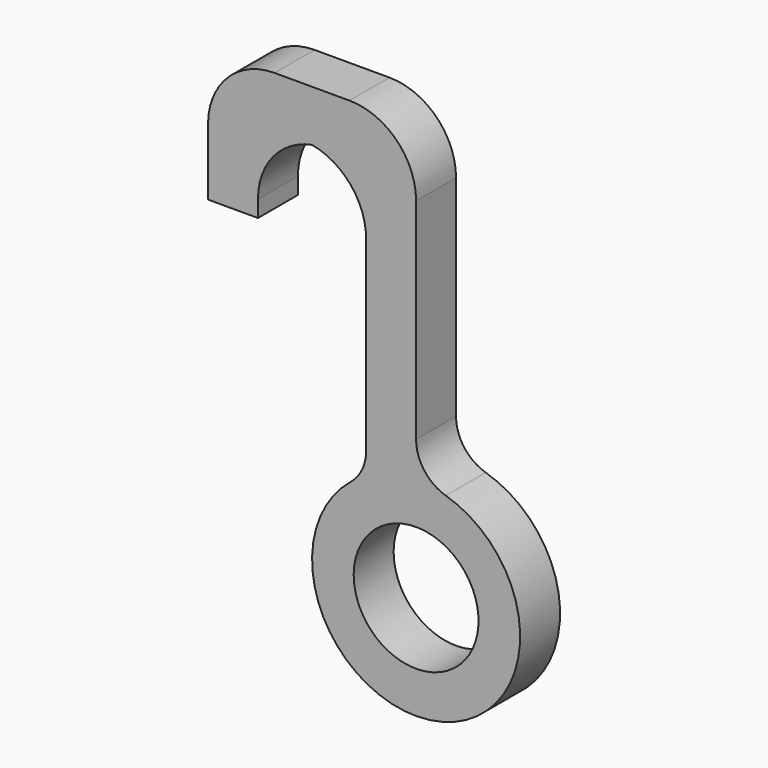
from build123d import *

# Parameters (mm, degrees)
F1_DEPTH    = 6
F2_R        = 12.5
F3_DEPTH    = 6
F5_D        = 15
F6_T1_DEPTH = 6
F6_T3_DEPTH = 46
F7_R        = 5


# Not quite as in the source:
# - a fillet or chamfer that OpenCascade refuses, or shapes differently, is made with other operations: its cross-section is extruded or revolved along the edge and cut away or added


with BuildPart() as f1:
    # F0 (on Front) → F1 (new body)
    with BuildSketch(Plane.XZ):
        Polygon((0, 0), (0, 40), (-25, 40), (-25, 24), (-19, 24), (-19, 34), (-6, 34), (-6, 0), align=None)
    extrude(amount=F1_DEPTH)

    # F2 (on Front) → F3 (join)
    with BuildSketch(Plane.XZ):
        with Locations((0, -10)):
            Circle(F2_R)
    extrude(amount=F3_DEPTH)

    # F5 (through all)
    with Locations(Plane.XZ.offset(6)):
        with Locations((0, -10)):
            Hole(F5_D / 2)

    # F6: fillet of radius 8 on 4 edges, made by hand

    # F6_s2 → F6_t1 (join)
    with BuildSketch(Plane.XZ):
        with BuildLine():
            ThreePointArc((-6, 26), (-8.3431457505, 31.6568542495), (-14, 34))
            Line((-14, 34), (-6, 34))
            Line((-6, 34), (-6, 26))
        make_face()
        with BuildLine():
            ThreePointArc((-11, 34), (-16.6568542495, 31.6568542495), (-19, 26))
            Line((-19, 26), (-19, 34))
            Line((-19, 34), (-11, 34))
        make_face()
    extrude(amount=F6_T1_DEPTH)

    # F6_s4 → F6_t3 (cut)
    with BuildSketch(Plane.XZ.offset(-20)):
        with BuildLine():
            ThreePointArc((0, 32), (-2.3431457505, 37.6568542495), (-8, 40))
            Line((-8, 40), (0, 40))
            Line((0, 40), (0, 32))
        make_face()
        with BuildLine():
            ThreePointArc((-17, 40), (-22.6568542495, 37.6568542495), (-25, 32))
            Line((-25, 32), (-25, 40))
            Line((-25, 40), (-17, 40))
        make_face()
    extrude(amount=F6_T3_DEPTH, mode=Mode.SUBTRACT)

    # F7
    f7_edges = [f1.edges().sort_by_distance(p)[0] for p in [
        (-6, -3, 0.965856),
        (0, -3, 2.5),
    ]]
    fillet(f7_edges, radius=F7_R)


solid = f1.part
